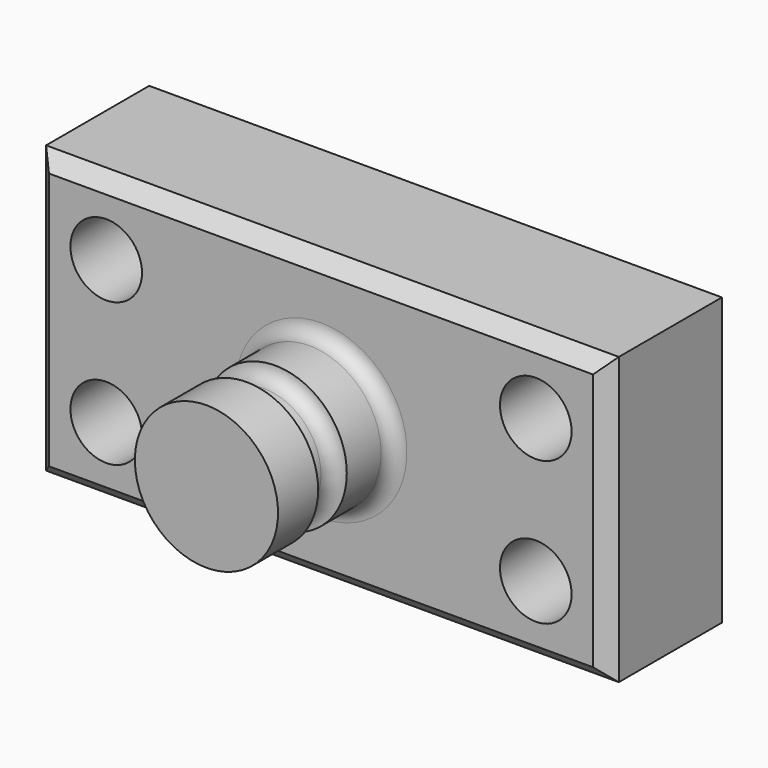
from build123d import *

# Parameters (mm, degrees)
F0_W     = 101.6
F0_H     = 50.8
F1_DEPTH = 25.4
F2_R     = 6.35
F3_DEPTH = 25.401
F4_W     = 12.7
F4_H     = 25.4
F6_W     = 12.0790981405
F6_H     = 6.35
F8_R     = 2.53999
F9_SIZE  = 2.54


# Not quite as in the source:
# - a fillet or chamfer is up to 0.001 mm smaller than in the source, because OpenCascade refuses the exact size


with BuildPart() as f1:
    # F0 (on Front) → F1 (new body)
    with BuildSketch(Plane.XZ):
        Rectangle(F0_W, F0_H)
    extrude(amount=F1_DEPTH)

    # F2 (on face) → F3 (cut, through all)
    with BuildSketch(Plane.XZ.offset(25.4)):
        with Locations((-38.1, 12.7)):
            Circle(F2_R)
        with Locations((-38.1, -12.7)):
            Circle(F2_R)
        with Locations((38.1, 12.7)):
            Circle(F2_R)
        with Locations((38.1, -12.7)):
            Circle(F2_R)
    extrude(amount=-F3_DEPTH, mode=Mode.SUBTRACT)

    # F4 (on Top) → F5 (revolve)
    with BuildSketch(Plane.XY):
        with Locations((-6.35, -38.1)):
            Rectangle(F4_W, F4_H)
    revolve(axis=Axis((0, -38.1, 0), (0, -1, 0)))

    # F6 (on Top) → F7 (revolve, cut)
    with BuildSketch(Plane.XY):
        with Locations((16.1995490702, -38.735)):
            Rectangle(F6_W, F6_H)
    revolve(axis=Axis((0, -40.3367578983, 0), (0, -1, 0)), mode=Mode.SUBTRACT)

    # F8 (radius 2.54 in the source; OpenCascade refuses exactly that, so slightly less here)
    f8_edges = [f1.edges().sort_by_distance(p)[0] for p in [
        (12.7, -25.4, 0),
        (-10.16, -41.91, 0),
        (-10.16, -35.56, 0),
    ]]
    fillet(f8_edges, radius=F8_R)

    # F9
    f9_edges = [f1.edges().sort_by_distance(p)[0] for p in [
        (0, -25.4, 25.4),
        (-50.8, -25.4, 0),
        (0, -25.4, -25.4),
        (50.8, -25.4, 0),
    ]]
    chamfer(f9_edges, length=F9_SIZE)


solid = f1.part
